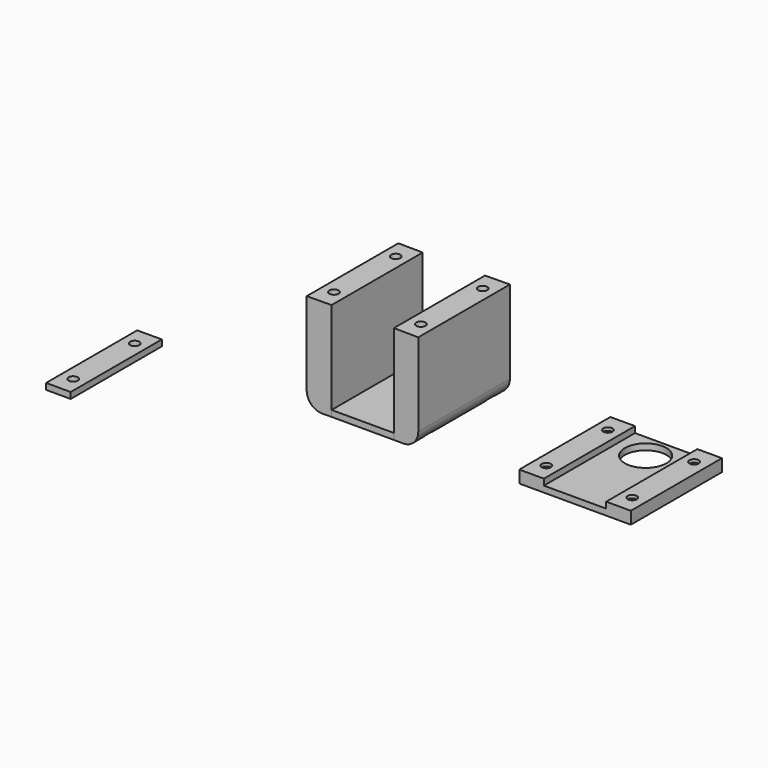
from build123d import *

# Parameters (mm, degrees)
F0_W         = 20.25
F0_H         = 37
F0_R         = 6.75
F1_DEPTH     = 2
F0_R_2       = 1.5
F2_DEPTH     = 32
F3_DEPTH     = 29
F4_W         = 20.25
F4_H         = 37
F4_R         = 6.75
F5_DEPTH     = 2
F6_W         = 8
F6_H         = 37
F6_R         = 1.5
F7_DEPTH     = 2
F4_W_2       = 8
F4_R_2       = 1.5
F8_DEPTH     = 4
F9_DEPTH     = 3
F10_T1_DEPTH = 62.2068632793


# Not quite as in the source:
# - a fillet or chamfer that OpenCascade refuses, or shapes differently, is made with other operations: its cross-section is extruded or revolved along the edge and cut away or added


with BuildPart() as f1:
    # F0 (on Top) → F1 (new body)
    with BuildSketch(Plane.XY):
        Rectangle(F0_W, F0_H)
        with Locations((0, 10.5)):
            Circle(F0_R, mode=Mode.SUBTRACT)
    extrude(amount=F1_DEPTH)

    # F0 (on Top) → F2 (join)
    with BuildSketch(Plane.XY):
        Polygon((-10.125, -18.5), (-10.125, 18.5), (-18.125, 18.6034316397), (-18.125, -18.6034316397), align=None)
        Polygon((-16.6148230359, -11.1137143672), (-14.125, -9.6762143672), (-11.6351769641, -11.1137143672), (-11.6351769641, -13.9887143672), (-14.125, -15.4262143672), (-16.6148230359, -13.9887143672), align=None, mode=Mode.SUBTRACT)
        Polygon((-17, 14.2110963911), (-14.125, 15.870978415), (-11.25, 14.2110963911), (-11.25, 10.8913323432), (-14.125, 9.2314503193), (-17, 10.8913323432), align=None, mode=Mode.SUBTRACT)
        Polygon((18.125, 18.6034316397), (10.125, 18.5), (10.125, -18.5), (18.125, -18.6034316397), align=None)
        Polygon((11.25, -10.8913323432), (14.125, -9.2314503193), (17, -10.8913323432), (17, -14.2110963911), (14.125, -15.870978415), (11.25, -14.2110963911), align=None, mode=Mode.SUBTRACT)
        Polygon((11.25, 14.2110963911), (14.125, 15.870978415), (17, 14.2110963911), (17, 10.8913323432), (14.125, 9.2314503193), (11.25, 10.8913323432), align=None, mode=Mode.SUBTRACT)
        Polygon((17, -10.8913323432), (14.125, -9.2314503193), (11.25, -10.8913323432), (11.25, -14.2110963911), (14.125, -15.870978415), (17, -14.2110963911), align=None)
        with Locations((14.125, -12.5512143672)):
            Circle(F0_R_2, mode=Mode.SUBTRACT)
        Polygon((-11.6351769641, -11.1137143672), (-14.125, -9.6762143672), (-16.6148230359, -11.1137143672), (-16.6148230359, -13.9887143672), (-14.125, -15.4262143672), (-11.6351769641, -13.9887143672), align=None)
        with Locations((-14.125, -12.5512143672)):
            Circle(F0_R_2, mode=Mode.SUBTRACT)
        Polygon((-11.25, 14.2110963911), (-14.125, 15.870978415), (-17, 14.2110963911), (-17, 10.8913323432), (-14.125, 9.2314503193), (-11.25, 10.8913323432), align=None)
        with Locations((-14.125, 12.5512143672)):
            Circle(F0_R_2, mode=Mode.SUBTRACT)
        Polygon((17, 14.2110963911), (14.125, 15.870978415), (11.25, 14.2110963911), (11.25, 10.8913323432), (14.125, 9.2314503193), (17, 10.8913323432), align=None)
        with Locations((14.125, 12.5512143672)):
            Circle(F0_R_2, mode=Mode.SUBTRACT)
    extrude(amount=F2_DEPTH)

    # F0 (on Top) → F3 (cut)
    with BuildSketch(Plane.XY):
        Polygon((17, -10.8913323432), (14.125, -9.2314503193), (11.25, -10.8913323432), (11.25, -14.2110963911), (14.125, -15.870978415), (17, -14.2110963911), align=None)
        with Locations((14.125, -12.5512143672)):
            Circle(F0_R_2, mode=Mode.SUBTRACT)
        Polygon((17, 14.2110963911), (14.125, 15.870978415), (11.25, 14.2110963911), (11.25, 10.8913323432), (14.125, 9.2314503193), (17, 10.8913323432), align=None)
        with Locations((14.125, 12.5512143672)):
            Circle(F0_R_2, mode=Mode.SUBTRACT)
        Polygon((-11.25, 14.2110963911), (-14.125, 15.870978415), (-17, 14.2110963911), (-17, 10.8913323432), (-14.125, 9.2314503193), (-11.25, 10.8913323432), align=None)
        with Locations((-14.125, 12.5512143672)):
            Circle(F0_R_2, mode=Mode.SUBTRACT)
        Polygon((-11.6351769641, -11.1137143672), (-14.125, -9.6762143672), (-16.6148230359, -11.1137143672), (-16.6148230359, -13.9887143672), (-14.125, -15.4262143672), (-11.6351769641, -13.9887143672), align=None)
        with Locations((-14.125, -12.5512143672)):
            Circle(F0_R_2, mode=Mode.SUBTRACT)
    extrude(amount=F3_DEPTH, mode=Mode.SUBTRACT)

    # F10: fillet of radius 5 on 2 edges, made by hand

    # F10_s2 → F10_t1 (cut)
    with BuildSketch(Plane.XZ.offset(-31.1034316397)):
        with BuildLine():
            ThreePointArc((-13.125, 0), (-16.6605339059, 1.4644660941), (-18.125, 5))
            Line((-18.125, 5), (-18.125, 0))
            Line((-18.125, 0), (-13.125, 0))
        make_face()
        with BuildLine():
            ThreePointArc((13.125, 0), (16.6605339059, 1.4644660941), (18.125, 5))
            Line((18.125, 5), (18.125, 0))
            Line((18.125, 0), (13.125, 0))
        make_face()
    extrude(amount=F10_T1_DEPTH, mode=Mode.SUBTRACT)


with BuildPart() as f5:
    # F4 (on Top) → F5 (new body)
    with BuildSketch(Plane.XY):
        with Locations((68.0498939753, 1.1739132404)):
            Rectangle(F4_W, F4_H)
        with Locations((67.7923956513, 11.6739132404)):
            Circle(F4_R, mode=Mode.SUBTRACT)
    extrude(amount=F5_DEPTH)

    # F4 (on Top) → F8 (join)
    with BuildSketch(Plane.XY):
        with Locations((53.9248939753, 1.1739132404)):
            Rectangle(F4_W_2, F4_H)
        Polygon((53.9248939753, -14.5015132401), (51.1748939753, -12.9137999998), (51.1748939753, -9.7383735193), (53.9248939753, -8.150660279), (56.6748939753, -9.7383735193), (56.6748939753, -12.9137999998), align=None, mode=Mode.SUBTRACT)
        Polygon((53.9248939753, 10.4984867599), (51.1748939753, 12.0862000002), (51.1748939753, 15.2616264807), (53.9248939753, 16.849339721), (56.6748939753, 15.2616264807), (56.6748939753, 12.0862000002), align=None, mode=Mode.SUBTRACT)
        with Locations((82.1748939753, 1.1739132404)):
            Rectangle(F4_W_2, F4_H)
        Polygon((81.9173956513, -8.2939509534), (84.6673956513, -9.8816641936), (84.6673956513, -13.0570906742), (81.9173956513, -14.6448039144), (79.1673956513, -13.0570906742), (79.1673956513, -9.8816641936), align=None, mode=Mode.SUBTRACT)
        Polygon((81.9173956513, 16.849339721), (84.6673956513, 15.2616264807), (84.6673956513, 12.0862000002), (81.9173956513, 10.4984867599), (79.1673956513, 12.0862000002), (79.1673956513, 15.2616264807), align=None, mode=Mode.SUBTRACT)
        Polygon((51.1748939753, -9.7383735193), (51.1748939753, -12.9137999998), (53.9248939753, -14.5015132401), (56.6748939753, -12.9137999998), (56.6748939753, -9.7383735193), (53.9248939753, -8.150660279), align=None)
        with Locations((53.9248939753, -11.3260867596)):
            Circle(F4_R_2, mode=Mode.SUBTRACT)
        Polygon((51.1748939753, 15.2616264807), (51.1748939753, 12.0862000002), (53.9248939753, 10.4984867599), (56.6748939753, 12.0862000002), (56.6748939753, 15.2616264807), (53.9248939753, 16.849339721), align=None)
        with Locations((53.9248939753, 13.6739132404)):
            Circle(F4_R_2, mode=Mode.SUBTRACT)
        Polygon((84.6673956513, -13.0570906742), (84.6673956513, -9.8816641936), (81.9173956513, -8.2939509534), (79.1673956513, -9.8816641936), (79.1673956513, -13.0570906742), (81.9173956513, -14.6448039144), align=None)
        with Locations((81.9173956513, -11.4693774339)):
            Circle(F4_R_2, mode=Mode.SUBTRACT)
        Polygon((84.6673956513, 12.0862000002), (84.6673956513, 15.2616264807), (81.9173956513, 16.849339721), (79.1673956513, 15.2616264807), (79.1673956513, 12.0862000002), (81.9173956513, 10.4984867599), align=None)
        with Locations((81.9173956513, 13.6739132404)):
            Circle(F4_R_2, mode=Mode.SUBTRACT)
    extrude(amount=F8_DEPTH)

    # F4 (on Top) → F9 (cut)
    with BuildSketch(Plane.XY):
        Polygon((51.1748939753, 15.2616264807), (51.1748939753, 12.0862000002), (53.9248939753, 10.4984867599), (56.6748939753, 12.0862000002), (56.6748939753, 15.2616264807), (53.9248939753, 16.849339721), align=None)
        with Locations((53.9248939753, 13.6739132404)):
            Circle(F4_R_2, mode=Mode.SUBTRACT)
        Polygon((84.6673956513, 12.0862000002), (84.6673956513, 15.2616264807), (81.9173956513, 16.849339721), (79.1673956513, 15.2616264807), (79.1673956513, 12.0862000002), (81.9173956513, 10.4984867599), align=None)
        with Locations((81.9173956513, 13.6739132404)):
            Circle(F4_R_2, mode=Mode.SUBTRACT)
        Polygon((84.6673956513, -13.0570906742), (84.6673956513, -9.8816641936), (81.9173956513, -8.2939509534), (79.1673956513, -9.8816641936), (79.1673956513, -13.0570906742), (81.9173956513, -14.6448039144), align=None)
        with Locations((81.9173956513, -11.4693774339)):
            Circle(F4_R_2, mode=Mode.SUBTRACT)
        Polygon((51.1748939753, -9.7383735193), (51.1748939753, -12.9137999998), (53.9248939753, -14.5015132401), (56.6748939753, -12.9137999998), (56.6748939753, -9.7383735193), (53.9248939753, -8.150660279), align=None)
        with Locations((53.9248939753, -11.3260867596)):
            Circle(F4_R_2, mode=Mode.SUBTRACT)
    extrude(amount=F9_DEPTH, mode=Mode.SUBTRACT)


with BuildPart() as f7:
    # F6 (on Top) → F7 (new body)
    with BuildSketch(Plane.XY):
        with Locations((-71.9763954457, -33.6543595721)):
            Rectangle(F6_W, F6_H)
        with Locations((-71.9763954457, -46.1543595721)):
            Circle(F6_R, mode=Mode.SUBTRACT)
        with Locations((-71.9763954457, -21.1543595721)):
            Circle(F6_R, mode=Mode.SUBTRACT)
    extrude(amount=F7_DEPTH)


solid = Compound([f1.part, f5.part, f7.part])
